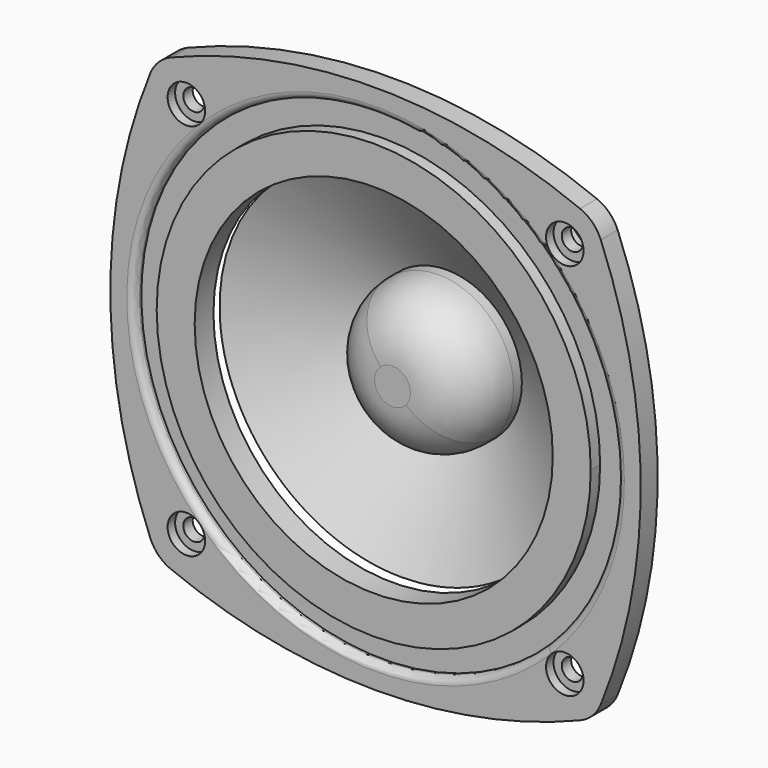
from build123d import *

# Parameters (mm, degrees)
F0_R     = 4
F1_DEPTH = 4.5
F2_R     = 1.49999
F3_DEPTH = 4.5
F4_DEPTH = 2.5
F5_DEPTH = 5
F6_DEPTH = 20
F8_DEPTH = 20
F9_DEPTH = 2.5
F0_R_2   = 2.25
F10_R    = 12.2
F11_R    = 8


# Not quite as in the source:
# - a fillet or chamfer that OpenCascade refuses, or shapes differently, is made with other operations: its cross-section is extruded or revolved along the edge and cut away or added
# - a fillet or chamfer is up to 0.001 mm smaller than in the source, because OpenCascade refuses the exact size


with BuildPart() as f1:
    # F0 (on Front) → F1 (new body)
    with BuildSketch(Plane.XZ):
        with BuildLine():
            ThreePointArc((46.6501257851, 46.6691146691), (-0.0189217732, 56.5000671107), (-46.6879693315, 46.6691146691))
            ThreePointArc((-46.6879693315, 46.6691146691), (-56.5, 6.71107e-05), (-46.6879693315, -46.6689804476))
            ThreePointArc((-46.6879693315, -46.6689804476), (-23.840882854, -54.0207126295), (0.0315038717, -56.4999218996))
            ThreePointArc((0.0315038717, -56.4999218996), (23.852382057, -54.010318455), (46.6501257851, -46.6689804476))
            ThreePointArc((46.6501257851, -46.6689804476), (56.4810782268, 6.71107e-05), (46.6501257851, 46.6691146691))
        make_face()
        with Locations((-40.3050865276, -40.3050865276)):
            Circle(F0_R, mode=Mode.SUBTRACT)
        with BuildLine():
            ThreePointArc((43.1240706101, -43.1429252727), (37.4766594029, -43.1335136524), (37.4672477826, -37.4861024452))
            ThreePointArc((37.4672477826, -37.4861024452), (41.8296594219, -36.6070225084), (44.3050865276, -40.3050865276))
            ThreePointArc((44.3050865276, -40.3050865276), (43.9980485048, -41.8419768409), (43.1240706101, -43.1429252727))
        make_face(mode=Mode.SUBTRACT)
        with BuildLine():
            ThreePointArc((-36.4254253421, 36.4065706796), (19.7020379007, 47.5823465432), (51.5, 0))
            ThreePointArc((51.5, 0), (47.5772445083, -19.7143553027), (36.4065706795, -36.4254253421))
            ThreePointArc((36.4065706795, -36.4254253421), (-36.4159992311, -36.4159992311), (-36.4254253421, 36.4065706796))
        make_face(mode=Mode.SUBTRACT)
        with BuildLine():
            ThreePointArc((-36.3050865276, 40.3050865276), (-36.6121245504, 38.7681962144), (-37.4861024451, 37.4672477827))
            ThreePointArc((-37.4861024451, 37.4672477827), (-43.1335136524, 37.4766594029), (-43.1429252726, 43.1240706102))
            ThreePointArc((-43.1429252726, 43.1240706102), (-38.7805136333, 44.0031505468), (-36.3050865276, 40.3050865276))
        make_face(mode=Mode.SUBTRACT)
        with Locations((40.3050865276, 40.3050865276)):
            Circle(F0_R, mode=Mode.SUBTRACT)
    extrude(amount=F1_DEPTH)

    # F2 (radius 1.5 in the source; OpenCascade refuses exactly that, so slightly less here)
    f2_edges = [f1.edges().sort_by_distance(p)[0] for p in [
        (-51.5, -4.5, 0),
    ]]
    fillet(f2_edges, radius=F2_R)

    # F11
    f11_edges = [f1.edges().sort_by_distance(p)[0] for p in [
        (-46.687969, -2.25, 46.669115),
        (46.650126, -2.25, 46.669115),
        (46.650126, -2.25, -46.66898),
        (-46.687969, -2.25, -46.66898),
    ]]
    fillet(f11_edges, radius=F11_R)


with BuildPart() as f3:
    # F0 (on Front) → F3 (new body)
    with BuildSketch(Plane.XZ):
        with BuildLine():
            Line((-32.6975760945, 32.678721432), (-36.4254253421, 36.4065706796))
            ThreePointArc((-36.4254253421, 36.4065706796), (-36.4159992311, -36.4159992311), (36.4065706795, -36.4254253421))
            Line((36.4065706795, -36.4254253421), (32.6787214319, -32.6975760945))
            ThreePointArc((32.6787214319, -32.6975760945), (-32.6881501227, -32.6881501226), (-32.6975760945, 32.678721432))
        make_face()
        with BuildLine():
            ThreePointArc((36.4065706795, -36.4254253421), (47.5772445083, -19.7143553027), (51.5, 0))
            ThreePointArc((51.5, 0), (19.7020379007, 47.5823465432), (-36.4254253421, 36.4065706796))
            Line((-36.4254253421, 36.4065706796), (-32.6975760945, 32.678721432))
            ThreePointArc((-32.6975760945, 32.678721432), (17.6845404825, 42.711676914), (46.2280252324, 0))
            ThreePointArc((46.2280252324, 0), (42.7065748791, -17.6968578845), (32.6787214319, -32.6975760945))
            Line((32.6787214319, -32.6975760945), (36.4065706795, -36.4254253421))
        make_face()
    extrude(amount=-F3_DEPTH)


with BuildPart() as f4:
    # F0 (on Front) → F4 (new body)
    with BuildSketch(Plane.XZ):
        with BuildLine():
            Line((-32.6975760945, 32.678721432), (-36.4254253421, 36.4065706796))
            ThreePointArc((-36.4254253421, 36.4065706796), (-36.4159992311, -36.4159992311), (36.4065706795, -36.4254253421))
            Line((36.4065706795, -36.4254253421), (32.6787214319, -32.6975760945))
            ThreePointArc((32.6787214319, -32.6975760945), (-32.6881501227, -32.6881501226), (-32.6975760945, 32.678721432))
        make_face()
        with BuildLine():
            ThreePointArc((36.4065706795, -36.4254253421), (47.5772445083, -19.7143553027), (51.5, 0))
            ThreePointArc((51.5, 0), (19.7020379007, 47.5823465432), (-36.4254253421, 36.4065706796))
            Line((-36.4254253421, 36.4065706796), (-32.6975760945, 32.678721432))
            ThreePointArc((-32.6975760945, 32.678721432), (17.6845404825, 42.711676914), (46.2280252324, 0))
            ThreePointArc((46.2280252324, 0), (42.7065748791, -17.6968578845), (32.6787214319, -32.6975760945))
            Line((32.6787214319, -32.6975760945), (36.4065706795, -36.4254253421))
        make_face()
    extrude(amount=F4_DEPTH)

    # F0 (on Front) → F5 (join)
    with BuildSketch(Plane.XZ):
        with BuildLine():
            Line((-26.9789756853, 26.9601210229), (-32.6975760945, 32.678721432))
            ThreePointArc((-32.6975760945, 32.678721432), (-32.6881501227, -32.6881501226), (32.6787214319, -32.6975760945))
            Line((32.6787214319, -32.6975760945), (26.9601210228, -26.9789756854))
            ThreePointArc((26.9601210228, -26.9789756854), (-26.9695500018, -26.9695500018), (-26.9789756853, 26.9601210229))
        make_face()
        with BuildLine():
            ThreePointArc((46.2280252324, 0), (17.6845404825, 42.711676914), (-32.6975760945, 32.678721432))
            Line((-32.6975760945, 32.678721432), (-26.9789756853, 26.9601210229))
            ThreePointArc((-26.9789756853, 26.9601210229), (14.5896563597, 35.239965691), (38.1407033836, 0))
            ThreePointArc((38.1407033836, 0), (35.234863656, -14.6019737618), (26.9601210228, -26.9789756854))
            Line((26.9601210228, -26.9789756854), (32.6787214319, -32.6975760945))
            ThreePointArc((32.6787214319, -32.6975760945), (42.7065748791, -17.6968578845), (46.2280252324, 0))
        make_face()
    extrude(amount=F5_DEPTH)


with BuildPart() as f6:
    # F0 (on Front) → F6 (new body)
    with BuildSketch(Plane.XZ):
        with BuildLine():
            Line((-10.6323599426, 10.6135052801), (-26.9789756853, 26.9601210229))
            ThreePointArc((-26.9789756853, 26.9601210229), (-26.9695500018, -26.9695500018), (26.9601210228, -26.9789756854))
            Line((26.9601210228, -26.9789756854), (11.9685153649, -11.9873700274))
            ThreePointArc((11.9685153649, -11.9873700274), (-11.3201686822, -12.675178767), (-10.6323599426, 10.6135052801))
        make_face()
        with BuildLine():
            ThreePointArc((38.1407033836, 0), (14.5896563597, 35.239965691), (-26.9789756853, 26.9601210229))
            Line((-26.9789756853, 26.9601210229), (-10.6323599426, 10.6135052801))
            ThreePointArc((-10.6323599426, 10.6135052801), (6.5603940746, 13.2481973565), (16.0091360787, -1.3550100848))
            ThreePointArc((16.0091360787, -1.3550100848), (14.9649261462, -7.0421379562), (11.9685153649, -11.9873700274))
            Line((11.9685153649, -11.9873700274), (26.9601210228, -26.9789756854))
            ThreePointArc((26.9601210228, -26.9789756854), (35.234863656, -14.6019737618), (38.1407033836, 0))
        make_face()
    extrude(amount=-F6_DEPTH)

    # F7: chamfer of 25 x 14.4337567297 on 1 edges, made by hand

    # F7_s1 → F7_t2 (revolve, cut)
    with BuildSketch(Plane(origin=(-0.6727855999, 0, -0.5976763571), x_dir=(0, 1, 0), z_dir=(-0.747605324, 0, -0.6641432673))):
        Polygon((14.4337567297, -14.9961233253), (0, -39.9961233253), (0, -14.9961233253), align=None)
    revolve(axis=Axis((0, 0, -1.3550100848), (0, 1, 0)), mode=Mode.SUBTRACT)


with BuildPart() as f8:
    # F0 (on Front) → F8 (new body)
    with BuildSketch(Plane.XZ):
        with BuildLine():
            Line((11.9685153649, -11.9873700274), (-10.6323599426, 10.6135052801))
            ThreePointArc((-10.6323599426, 10.6135052801), (-11.3201686822, -12.675178767), (11.9685153649, -11.9873700274))
        make_face()
        with BuildLine():
            ThreePointArc((16.0091360787, -1.3550100848), (6.5603940746, 13.2481973565), (-10.6323599426, 10.6135052801))
            Line((-10.6323599426, 10.6135052801), (11.9685153649, -11.9873700274))
            ThreePointArc((11.9685153649, -11.9873700274), (14.9649261462, -7.0421379562), (16.0091360787, -1.3550100848))
        make_face()
    extrude(amount=-F8_DEPTH)

    # F10
    f10_edges = [f8.edges().sort_by_distance(p)[0] for p in [
        (-11.968515, 0, 9.27735),
    ]]
    fillet(f10_edges, radius=F10_R)


with BuildPart() as f9:
    # F0 (on Front) → F9 (new body)
    with BuildSketch(Plane.XZ):
        with BuildLine():
            ThreePointArc((-43.1429252726, 43.1240706102), (-43.1335136524, 37.4766594029), (-37.4861024451, 37.4672477827))
            Line((-37.4861024451, 37.4672477827), (-38.723551532, 38.7046968696))
            ThreePointArc((-38.723551532, 38.7046968696), (-41.8960767853, 38.71409627), (-41.9054761857, 41.8866215233))
            Line((-41.9054761857, 41.8866215233), (-43.1429252726, 43.1240706102))
        make_face()
        with BuildLine():
            Line((-38.723551532, 38.7046968696), (-37.4861024451, 37.4672477827))
            ThreePointArc((-37.4861024451, 37.4672477827), (-36.6121245504, 38.7681962144), (-36.3050865276, 40.3050865276))
            ThreePointArc((-36.3050865276, 40.3050865276), (-38.7805136333, 44.0031505468), (-43.1429252726, 43.1240706102))
            Line((-43.1429252726, 43.1240706102), (-41.9054761857, 41.8866215233))
            ThreePointArc((-41.9054761857, 41.8866215233), (-39.4502113118, 42.3863573811), (-38.0550865276, 40.3050865276))
            ThreePointArc((-38.0550865276, 40.3050865276), (-38.2289177315, 39.4378938559), (-38.723551532, 38.7046968696))
        make_face()
    extrude(amount=F9_DEPTH)


with BuildPart() as f9b:
    # F0 (on Front) → F9, piece 2 (new body)
    with BuildSketch(Plane.XZ):
        with Locations((40.3050865276, 40.3050865276)):
            Circle(F0_R)
        with Locations((40.3050865276, 40.3050865276)):
            Circle(F0_R_2, mode=Mode.SUBTRACT)
    extrude(amount=F9_DEPTH)


with BuildPart() as f9c:
    # F0 (on Front) → F9, piece 3 (new body)
    with BuildSketch(Plane.XZ):
        with Locations((-40.3050865276, -40.3050865276)):
            Circle(F0_R)
        with Locations((-40.3050865276, -40.3050865276)):
            Circle(F0_R_2, mode=Mode.SUBTRACT)
    extrude(amount=F9_DEPTH)


with BuildPart() as f9d:
    # F0 (on Front) → F9, piece 4 (new body)
    with BuildSketch(Plane.XZ):
        with BuildLine():
            Line((38.7046968695, -38.7235515321), (37.4672477826, -37.4861024452))
            ThreePointArc((37.4672477826, -37.4861024452), (37.4766594029, -43.1335136524), (43.1240706101, -43.1429252727))
            Line((43.1240706101, -43.1429252727), (41.8866215232, -41.9054761858))
            ThreePointArc((41.8866215232, -41.9054761858), (38.71409627, -41.8960767853), (38.7046968695, -38.7235515321))
        make_face()
        with BuildLine():
            ThreePointArc((44.3050865276, -40.3050865276), (41.8296594219, -36.6070225084), (37.4672477826, -37.4861024452))
            Line((37.4672477826, -37.4861024452), (38.7046968695, -38.7235515321))
            ThreePointArc((38.7046968695, -38.7235515321), (41.1599617434, -38.2238156742), (42.5550865276, -40.3050865276))
            ThreePointArc((42.5550865276, -40.3050865276), (42.3812553238, -41.1722791994), (41.8866215232, -41.9054761858))
            Line((41.8866215232, -41.9054761858), (43.1240706101, -43.1429252727))
            ThreePointArc((43.1240706101, -43.1429252727), (43.9980485048, -41.8419768409), (44.3050865276, -40.3050865276))
        make_face()
    extrude(amount=F9_DEPTH)


solid = Compound([f1.part, f3.part, f4.part, f6.part, f8.part, f9.part, f9b.part, f9c.part, f9d.part])
